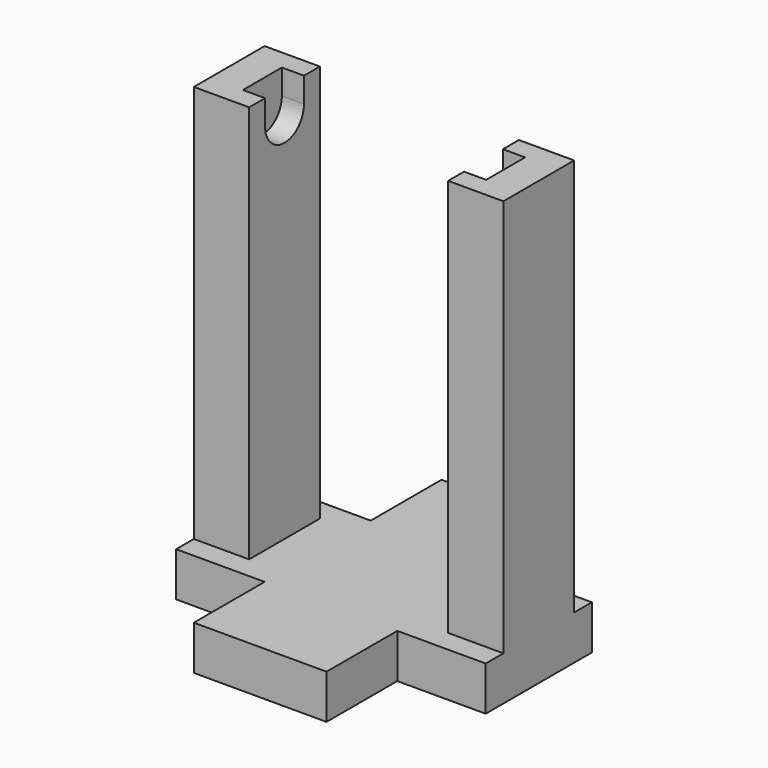
from build123d import *

# Parameters (mm, degrees)
F0_W     = 20
F0_H     = 30
F0_W_2   = 30
F0_H_2   = 20
F1_DEPTH = 10
F2_W     = 12.5
F2_H     = 20
F3_DEPTH = 100
F5_DEPTH = 27.5


with BuildPart() as f1:
    # F0 (on Top) → F1 (new body)
    with BuildSketch(Plane.XY):
        with Locations((25, 0)):
            Rectangle(F0_W, F0_H)
        with Locations((0, -25)):
            Rectangle(F0_W_2, F0_H_2)
        Rectangle(F0_W_2, F0_H)
        with Locations((-25, 0)):
            Rectangle(F0_W, F0_H)
        with Locations((0, 25)):
            Rectangle(F0_W_2, F0_H_2)
    extrude(amount=F1_DEPTH)

    # F2 (on Top) → F3 (join)
    with BuildSketch(Plane.XY):
        with Locations((-28.75, 0)):
            Rectangle(F2_W, F2_H)
        with Locations((28.75, 0)):
            Rectangle(F2_W, F2_H)
    extrude(amount=F3_DEPTH)

    # F4 (on Right) → F5 (cut, symmetric)
    with BuildSketch(Plane.YZ):
        with BuildLine():
            Line((-5.5, 100), (-5.5, 94.3625420332))
            ThreePointArc((-5.5, 94.3625420332), (0, 88.8625420332), (5.5, 94.3625420332))
            Line((5.5, 94.3625420332), (5.5, 100))
            Line((5.5, 100), (-5.5, 100))
        make_face()
    extrude(amount=F5_DEPTH, both=True, mode=Mode.SUBTRACT)


solid = f1.part
